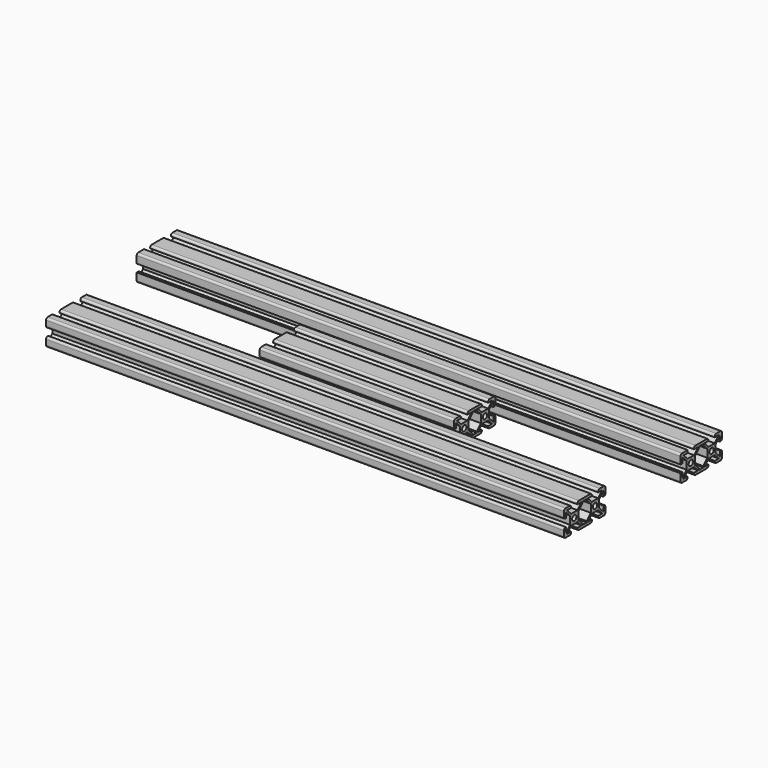
from build123d import *

# Parameters (mm, degrees)
F0_R          = 2.1
F1_DEPTH      = 75
F1_DEPTH_BACK = 75
F2_DEPTH      = 200
F2_DEPTH_BACK = 200
F3_DEPTH      = 210
F3_DEPTH_BACK = 210
F4_R          = 1.5
F4_2_R        = 1.5
F4_3_R        = 1.5


# Not quite as in the source:
# - a feature names something its author has since deleted; it is built from what else it names


with BuildPart() as f1:
    # F0 (on Right) → F1 (new body, two sides)
    with BuildSketch(Plane.YZ) as f1_sk:
        Polygon((-13.0807611845, 4), (-14, 4), (-14, 3.0807611845), (-14, -3.0807611845), (-14, -4), (-13.0807611845, -4), (-6.9192388155, -4), (-6, -4), (-6, -3.0807611845), (-6, 3.0807611845), (-6, 4), (-6.9192388155, 4), align=None)
        with Locations((-10, 0)):
            Circle(F0_R, mode=Mode.SUBTRACT)
        Polygon((6, 4), (6, 3.0807611845), (6, -3.0807611845), (6, -4), (6.9192388155, -4), (13.0807611845, -4), (14, -4), (14, -3.0807611845), (14, 3.0807611845), (14, 4), (13.0807611845, 4), (6.9192388155, 4), align=None)
        with Locations((10, 0)):
            Circle(F0_R, mode=Mode.SUBTRACT)
        Polygon((-14, 3.0807611845), (-14, 4), (-13.0807611845, 4), (-17.0807611845, 8), (-13, 8), (-13, 10), (-20, 10), (-20, 3), (-18, 3), (-18, 7.0807611845), align=None)
        Polygon((-14, -4), (-14, -3.0807611845), (-18, -7.0807611845), (-18, -3), (-20, -3), (-20, -10), (-13, -10), (-13, -8), (-17.0807611845, -8), (-13.0807611845, -4), align=None)
        Polygon((-2, -7.0807611845), (-6, -3.0807611845), (-6, -4), (-6.9192388155, -4), (-2.9192388155, -8), (-7, -8), (-7, -10), (7, -10), (7, -8), (2.9192388155, -8), (6.9192388155, -4), (6, -4), (6, -3.0807611845), (2, -7.0807611845), (2, -8), (-2.0242133178, -8), align=None)
        Polygon((-2.9192388155, 8), (-6.9192388155, 4), (-6, 4), (-6, 3.0807611845), (-2, 7.0807611845), (-2, 8), (2, 8), (2, 7.0807611845), (6, 3.0807611845), (6, 4), (6.9192388155, 4), (2.9192388155, 8), (7, 8), (7, 10), (-7, 10), (-7, 8), align=None)
        Polygon((20, 10), (13, 10), (13, 8), (17.0807611845, 8), (13.0807611845, 4), (14, 4), (14, 3.0807611845), (18, 7.0807611845), (18, 3), (20, 3), align=None)
        Polygon((20, -10), (20, -3), (18, -3), (18, -7.0807611845), (14, -3.0807611845), (14, -4), (13.0807611845, -4), (17.0807611845, -8), (13, -8), (13, -10), align=None)
    extrude(amount=F1_DEPTH)
    extrude(f1_sk.sketch, amount=-F1_DEPTH_BACK)

    # F4
    f4_edges = [f1.edges().sort_by_distance(p)[0] for p in [
        (0, 20, 10),
        (0, 7, 10),
        (0, 13, 10),
        (0, -7, 10),
        (0, -13, 10),
        (0, -20, 10),
        (0, -20, 3),
        (0, -20, -3),
        (0, -20, -10),
        (0, -13, -10),
        (0, -7, -10),
        (0, 7, -10),
        (0, 20, -10),
        (0, 20, -3),
        (0, 20, 3),
        (0, 13, -10),
    ]]
    fillet(f4_edges, radius=F4_R)


with BuildPart() as f2:
    # F0 (on Right) → F2 (new body, two sides)
    with BuildSketch(Plane.YZ) as f2_sk:
        Polygon((-14, 3.0807611845), (-14, 4), (-13.0807611845, 4), (-17.0807611845, 8), (-13, 8), (-13, 10), (-20, 10), (-20, 3), (-18, 3), (-18, 7.0807611845), align=None)
        Polygon((-13.0807611845, 4), (-14, 4), (-14, 3.0807611845), (-14, -3.0807611845), (-14, -4), (-13.0807611845, -4), (-6.9192388155, -4), (-6, -4), (-6, -3.0807611845), (-6, 3.0807611845), (-6, 4), (-6.9192388155, 4), align=None)
        with Locations((-10, 0)):
            Circle(F0_R, mode=Mode.SUBTRACT)
        Polygon((-14, -4), (-14, -3.0807611845), (-18, -7.0807611845), (-18, -3), (-20, -3), (-20, -10), (-13, -10), (-13, -8), (-17.0807611845, -8), (-13.0807611845, -4), align=None)
        Polygon((-2, -7.0807611845), (-6, -3.0807611845), (-6, -4), (-6.9192388155, -4), (-2.9192388155, -8), (-7, -8), (-7, -10), (7, -10), (7, -8), (2.9192388155, -8), (6.9192388155, -4), (6, -4), (6, -3.0807611845), (2, -7.0807611845), (2, -8), (-2.0242133178, -8), align=None)
        Polygon((-2.9192388155, 8), (-6.9192388155, 4), (-6, 4), (-6, 3.0807611845), (-2, 7.0807611845), (-2, 8), (2, 8), (2, 7.0807611845), (6, 3.0807611845), (6, 4), (6.9192388155, 4), (2.9192388155, 8), (7, 8), (7, 10), (-7, 10), (-7, 8), align=None)
        Polygon((20, 10), (13, 10), (13, 8), (17.0807611845, 8), (13.0807611845, 4), (14, 4), (14, 3.0807611845), (18, 7.0807611845), (18, 3), (20, 3), align=None)
        Polygon((20, -10), (20, -3), (18, -3), (18, -7.0807611845), (14, -3.0807611845), (14, -4), (13.0807611845, -4), (17.0807611845, -8), (13, -8), (13, -10), align=None)
        Polygon((6, 4), (6, 3.0807611845), (6, -3.0807611845), (6, -4), (6.9192388155, -4), (13.0807611845, -4), (14, -4), (14, -3.0807611845), (14, 3.0807611845), (14, 4), (13.0807611845, 4), (6.9192388155, 4), align=None)
        with Locations((10, 0)):
            Circle(F0_R, mode=Mode.SUBTRACT)
    extrude(amount=F2_DEPTH)
    extrude(f2_sk.sketch, amount=-F2_DEPTH_BACK)

    # F4#3
    f4_3_edges = [f2.edges().sort_by_distance(p)[0] for p in [
        (0, 20, 10),
        (0, 7, 10),
        (0, 13, 10),
        (0, -7, 10),
        (0, -13, 10),
        (0, -20, 10),
        (0, -20, 3),
        (0, -20, -3),
        (0, -20, -10),
        (0, -13, -10),
        (0, -7, -10),
        (0, 7, -10),
        (0, 20, -10),
        (0, 20, -3),
        (0, 20, 3),
        (0, 13, -10),
    ]]
    fillet(f4_3_edges, radius=F4_3_R)


with BuildPart() as f3:
    # F0 (on Right) → F3 (new body, two sides)
    with BuildSketch(Plane.YZ) as f3_sk:
        Polygon((-14, 3.0807611845), (-14, 4), (-13.0807611845, 4), (-17.0807611845, 8), (-13, 8), (-13, 10), (-20, 10), (-20, 3), (-18, 3), (-18, 7.0807611845), align=None)
        Polygon((-13.0807611845, 4), (-14, 4), (-14, 3.0807611845), (-14, -3.0807611845), (-14, -4), (-13.0807611845, -4), (-6.9192388155, -4), (-6, -4), (-6, -3.0807611845), (-6, 3.0807611845), (-6, 4), (-6.9192388155, 4), align=None)
        with Locations((-10, 0)):
            Circle(F0_R, mode=Mode.SUBTRACT)
        Polygon((-14, -4), (-14, -3.0807611845), (-18, -7.0807611845), (-18, -3), (-20, -3), (-20, -10), (-13, -10), (-13, -8), (-17.0807611845, -8), (-13.0807611845, -4), align=None)
        Polygon((-2, -7.0807611845), (-6, -3.0807611845), (-6, -4), (-6.9192388155, -4), (-2.9192388155, -8), (-7, -8), (-7, -10), (7, -10), (7, -8), (2.9192388155, -8), (6.9192388155, -4), (6, -4), (6, -3.0807611845), (2, -7.0807611845), (2, -8), (-2.0242133178, -8), align=None)
        Polygon((-2.9192388155, 8), (-6.9192388155, 4), (-6, 4), (-6, 3.0807611845), (-2, 7.0807611845), (-2, 8), (2, 8), (2, 7.0807611845), (6, 3.0807611845), (6, 4), (6.9192388155, 4), (2.9192388155, 8), (7, 8), (7, 10), (-7, 10), (-7, 8), align=None)
        Polygon((20, 10), (13, 10), (13, 8), (17.0807611845, 8), (13.0807611845, 4), (14, 4), (14, 3.0807611845), (18, 7.0807611845), (18, 3), (20, 3), align=None)
        Polygon((20, -10), (20, -3), (18, -3), (18, -7.0807611845), (14, -3.0807611845), (14, -4), (13.0807611845, -4), (17.0807611845, -8), (13, -8), (13, -10), align=None)
        Polygon((6, 4), (6, 3.0807611845), (6, -3.0807611845), (6, -4), (6.9192388155, -4), (13.0807611845, -4), (14, -4), (14, -3.0807611845), (14, 3.0807611845), (14, 4), (13.0807611845, 4), (6.9192388155, 4), align=None)
        with Locations((10, 0)):
            Circle(F0_R, mode=Mode.SUBTRACT)
    extrude(amount=F3_DEPTH)
    extrude(f3_sk.sketch, amount=-F3_DEPTH_BACK)

    # F4#2
    f4_2_edges = [f3.edges().sort_by_distance(p)[0] for p in [
        (0, 20, 10),
        (0, 7, 10),
        (0, 13, 10),
        (0, -7, 10),
        (0, -20, 10),
        (0, -20, -10),
        (0, -13, -10),
        (0, -7, -10),
        (0, 7, -10),
        (0, 20, -10),
        (0, 20, -3),
        (0, 20, 3),
        (0, 13, -10),
    ]]
    fillet(f4_2_edges, radius=F4_2_R)


with BuildPart() as f3_1:
    # F5: moved
    add(f3.part.moved(Location((0, 50, 0))))


with BuildPart() as f2_1:
    # F6: moved
    add(f2.part.moved(Location((0, -50, 0))))


solid = Compound([f1.part, f3_1.part, f2_1.part])
